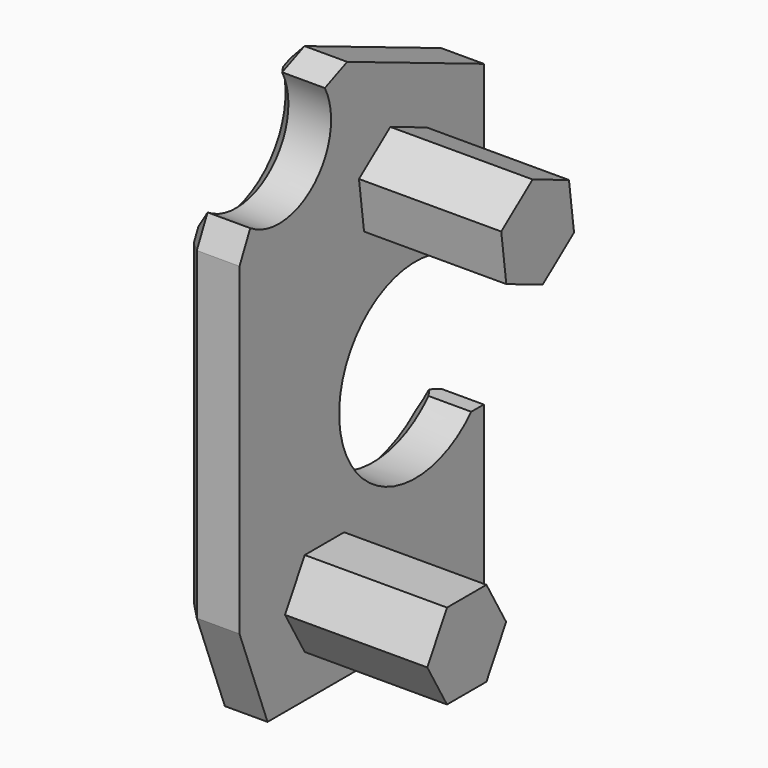
from build123d import *

# Parameters (mm, degrees)
F1_DEPTH    = 2
F2_DEPTH    = 5
F3_C1_SIZE  = 0.5
F3_C2_SIZE  = 0.5
F3_C3_SIZE  = 0.5
F3_C4_SIZE  = 0.5
F3_C5_SIZE  = 0.5
F3_C6_SIZE  = 0.5
F3_C7_SIZE  = 0.5
F3_C8_SIZE  = 0.5
F3_C9_SIZE  = 0.5
F3_C10_SIZE = 0.5


with BuildPart() as f1:
    # F0 (on Right) → F1 (new body)
    with BuildSketch(Plane.YZ):
        with BuildLine():
            Line((4.6591372722, 1.30894838), (5.2096475294, 1.30894838))
            Line((5.2096475294, 1.30894838), (5.2096475294, 7.2676605325))
            Line((5.2096475294, 7.2676605325), (-0.7903524706, 9.7676605325))
            Line((-0.7903524706, 9.7676605325), (-1.7747698447, 9.3573516256))
            ThreePointArc((-1.7747698447, 9.3573516256), (-2.2419413153, 6.578748784), (-5.0505708614, 6.3540645439))
            Line((-5.0505708614, 6.3540645439), (-5.5224032781, 5.3671410452))
            Line((-5.5224032781, 5.3671410452), (-5.5224032781, -6.0076899798))
            Line((-5.5224032781, -6.0076899798), (-4.2903524706, -9.2323394675))
            Line((-4.2903524706, -9.2323394675), (5.2096475294, -9.2323394675))
            Line((5.2096475294, -9.2323394675), (5.2096475294, -3.273627315))
            Line((5.2096475294, -3.273627315), (4.6591372722, -3.273627315))
            ThreePointArc((4.6591372722, -3.273627315), (-1.1444544368, -0.9823394675), (4.6591372722, 1.30894838))
        make_face()
        Polygon((-0.058301663, -6.2323394675), (-0.9243270668, -7.7323394675), (-2.6563778744, -7.7323394675), (-3.5224032781, -6.2323394675), (-2.6563778744, -4.7323394675), (-0.9243270668, -4.7323394675), align=None, mode=Mode.SUBTRACT)
        Polygon((-0.2736675582, 5.93383392), (1.1026635838, 6.9853626109), (2.7014797138, 6.3191892234), (2.9239647019, 4.601487145), (1.54763356, 3.5499584541), (-0.0511825701, 4.2161318417), align=None, mode=Mode.SUBTRACT)
        Polygon((-2.6563778744, -7.7323394675), (-0.9243270668, -7.7323394675), (-0.058301663, -6.2323394675), (-0.9243270668, -4.7323394675), (-2.6563778744, -4.7323394675), (-3.5224032781, -6.2323394675), align=None)
        Polygon((2.7014797138, 6.3191892234), (1.1026635838, 6.9853626109), (-0.2736675582, 5.93383392), (-0.0511825701, 4.2161318417), (1.54763356, 3.5499584541), (2.9239647019, 4.601487145), align=None)
    extrude(amount=-F1_DEPTH)

    # F0 (on Right) → F2 (join)
    with BuildSketch(Plane.YZ):
        Polygon((2.7014797138, 6.3191892234), (1.1026635838, 6.9853626109), (-0.2736675582, 5.93383392), (-0.0511825701, 4.2161318417), (1.54763356, 3.5499584541), (2.9239647019, 4.601487145), align=None)
        Polygon((-2.6563778744, -7.7323394675), (-0.9243270668, -7.7323394675), (-0.058301663, -6.2323394675), (-0.9243270668, -4.7323394675), (-2.6563778744, -4.7323394675), (-3.5224032781, -6.2323394675), align=None)
    extrude(amount=F2_DEPTH)

    # F3: chamfer of 0.5 on 12 edges, made by hand

    # F3_c1
    f3_c1_edges = [f1.edges().sort_by_distance(p)[0] for p in [
        (-2, -1.1444544368, -0.9823394675),
    ]]
    chamfer(f3_c1_edges, length=F3_C1_SIZE)

    # F3_c2
    f3_c2_edges = [f1.edges().sort_by_distance(p)[0] for p in [
        (-2, 5.2096475294, 4.352423109),
    ]]
    chamfer(f3_c2_edges, length=F3_C2_SIZE)

    # F3_c3
    f3_c3_edges = [f1.edges().sort_by_distance(p)[0] for p in [
        (-2, 1.9596475294, 8.6218271992),
    ]]
    chamfer(f3_c3_edges, length=F3_C3_SIZE)

    # F3_c4
    f3_c4_edges = [f1.edges().sort_by_distance(p)[0] for p in [
        (-2, -1.6075076826, 9.4270671311),
    ]]
    chamfer(f3_c4_edges, length=F3_C4_SIZE)

    # F3_c5
    f3_c5_edges = [f1.edges().sort_by_distance(p)[0] for p in [
        (-2, -2.43546855, 6.4198809023),
    ]]
    chamfer(f3_c5_edges, length=F3_C5_SIZE)

    # F3_c6
    f3_c6_edges = [f1.edges().sort_by_distance(p)[0] for p in [
        (-2, -5.39514647, 5.633321854),
    ]]
    chamfer(f3_c6_edges, length=F3_C6_SIZE)

    # F3_c7
    f3_c7_edges = [f1.edges().sort_by_distance(p)[0] for p in [
        (-2, -5.5224032781, -0.8998828859),
    ]]
    chamfer(f3_c7_edges, length=F3_C7_SIZE)

    # F3_c8
    f3_c8_edges = [f1.edges().sort_by_distance(p)[0] for p in [
        (-2, -4.6563778744, -8.2743403139),
    ]]
    chamfer(f3_c8_edges, length=F3_C8_SIZE)

    # F3_c9
    f3_c9_edges = [f1.edges().sort_by_distance(p)[0] for p in [
        (-2, 0.7272736227, -9.2323394675),
    ]]
    chamfer(f3_c9_edges, length=F3_C9_SIZE)

    # F3_c10
    f3_c10_edges = [f1.edges().sort_by_distance(p)[0] for p in [
        (-2, 5.2096475294, -6.067102044),
    ]]
    chamfer(f3_c10_edges, length=F3_C10_SIZE)


solid = f1.part
